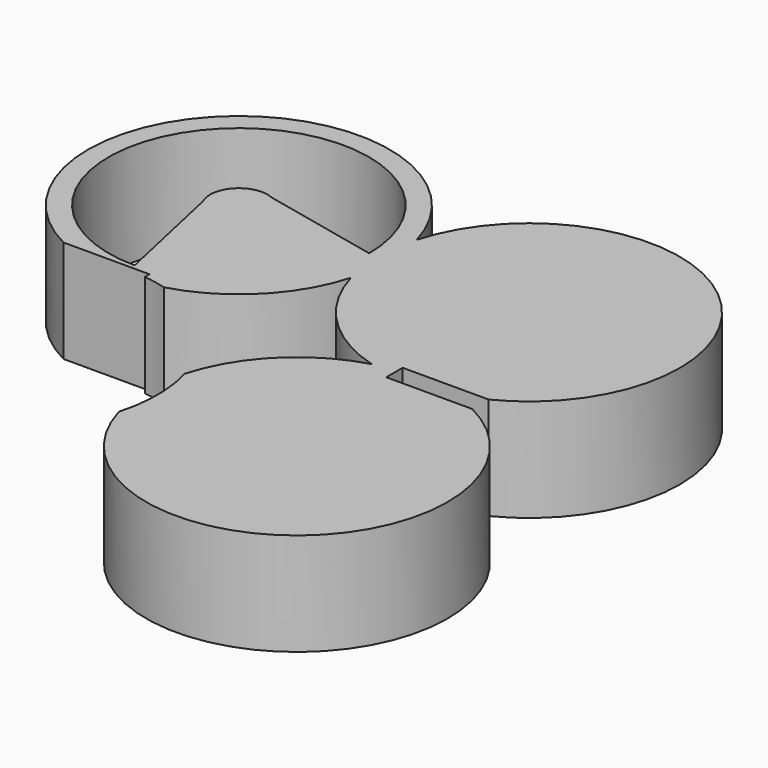
from build123d import *

# Parameters (mm, degrees)
F2_DEPTH = 25


# Not quite as in the source:
# - ends of sketch curves that miss each other by under 0.0002 mm in the source are joined


with BuildPart() as f2:
    # F1 (on face) → F2 (new body)
    with BuildSketch(Plane.XY):
        with BuildLine():
            ThreePointArc((-30.855476, 1.1181271498), (-28.0698825324, 0.6652748768), (-25.3272532308, 0))
            ThreePointArc((-25.3272532308, 0), (-9.3691647914, 9.3691647914), (0, 25.3272532308))
            ThreePointArc((0, 25.3272532308), (9.3691647914, 9.3691647914), (25.3272532308, 0))
            ThreePointArc((25.3272532308, 0), (9.3691647914, -9.3691647914), (0, -25.3272532308))
            ThreePointArc((0, -25.3272532308), (1.394661, -35.355339), (0, -45.3834247692))
            ThreePointArc((0, -45.3834247692), (58.7852402391, -63.6679197359), (51.8201256429, -2.5))
            Line((51.8201256429, -2.5), (30.855475, -2.5))
            Line((30.855475, -2.5), (30.855475, 2.5))
            Line((30.855475, 2.5), (51.8201256429, 2.5))
            ThreePointArc((51.8201256429, 2.5), (58.7852402391, 63.6679197359), (0, 45.3834247692))
            ThreePointArc((0, 45.3834247692), (-58.7852402391, 63.6679197359), (-51.8201256429, 2.5))
            Line((-51.8201256429, 2.5), (-30.855476, 2.5))
            Line((-30.855476, 2.5), (-30.855476, 1.1181271498))
        make_face()
        with BuildLine():
            ThreePointArc((-35.355339, 3.605339), (-57.8059793027, 57.8059793027), (-3.605339, 35.355339))
            Line((-3.605339, 35.355339), (-32.426206, 41.713026))
            ThreePointArc((-32.426206, 41.713026), (-40.3050867894, 40.3050861472), (-41.7130253526, 32.4262052983))
            Line((-41.7130253526, 32.4262052983), (-35.355339, 3.605339))
        make_face(mode=Mode.SUBTRACT)
    extrude(amount=F2_DEPTH)


solid = f2.part
